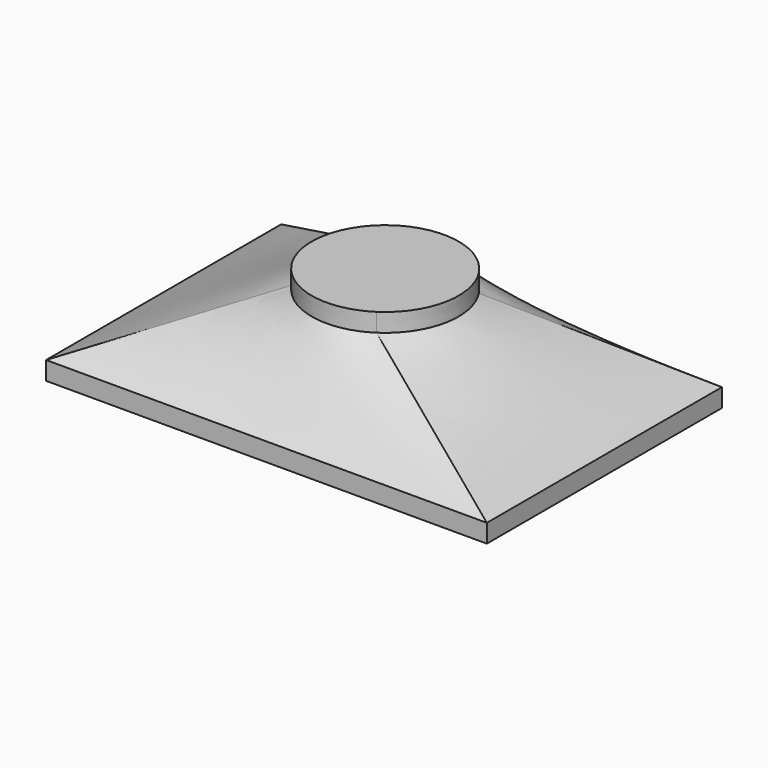
from build123d import *

# Parameters (mm, degrees)
F0_W      = 914.4
F0_H      = 609.6
F1_DEPTH  = 38.1
F1_FACE_W = 914.4
F1_FACE_H = 609.6
F5_DEPTH  = 38.1


# Not quite as in the source:
# - the arcs of a loft's sections are written as splines that run evenly, so that the points pair up as in the source's solid


with BuildPart() as f1:
    # F0 (on Top) → F1 (new body)
    with BuildSketch(Plane.XY):
        with Locations((0, -3.0270647792)):
            Rectangle(F0_W, F0_H)
    extrude(amount=F1_DEPTH)

    # F1_face (on face) → F4 section 0
    with BuildSketch(Plane(origin=(0, -3.0270647792, 38.1), x_dir=(1, 0, 0), z_dir=(0, 0, 1))):
        Rectangle(F1_FACE_W, F1_FACE_H)
    # F3 (on offset) → F4 section 1
    with BuildSketch(Plane.XY.offset(190.5)):
        with BuildLine():
            add(Edge.make_bspline(
                [(127.1917959248, 83.9524094319), (121.6971235765, 92.2770930084), (115.3826976006, 100.0604061319), (101.3563796815, 114.245945568), (93.6448345666, 120.6478211153), (77.1205669567, 131.8243905093), (68.3082530567, 136.5988079933), (49.9210540934, 144.3368980513), (40.3466236897, 147.3003792857), (20.8031031174, 151.3026195462), (10.8344962009, 152.3412796091), (-9.1142994449, 152.4538662235), (-19.0939949009, 151.5277899911), (-38.6814445909, 147.7463963189), (-48.2887144867, 144.8911723815), (-66.7620835141, 137.3611152609), (-75.6277258553, 132.6864682732), (-83.9524094319, 127.1917959248)],
                knots=[0, 0, 0, 0, 0.125, 0.125, 0.25, 0.25, 0.375, 0.375, 0.5, 0.5, 0.625, 0.625, 0.75, 0.75, 0.875, 0.875, 1, 1, 1, 1], degree=3))
            add(Edge.make_bspline(
                [(-83.9524094319, 127.1917959248), (-92.2770930084, 121.6971235765), (-100.0604061319, 115.3826976006), (-114.245945568, 101.3563796815), (-120.6478211153, 93.6448345666), (-131.8243905093, 77.1205669567), (-136.5988079933, 68.3082530567), (-144.3368980513, 49.9210540934), (-147.3003792857, 40.3466236897), (-151.3026195462, 20.8031031174), (-152.3412796091, 10.8344962009), (-152.4538662235, -9.1142994449), (-151.5277899911, -19.0939949009), (-147.7463963189, -38.6814445909), (-144.8911723815, -48.2887144867), (-137.3611152609, -66.7620835141), (-132.6864682732, -75.6277258553), (-127.1917959248, -83.9524094319)],
                knots=[0, 0, 0, 0, 0.125, 0.125, 0.25, 0.25, 0.375, 0.375, 0.5, 0.5, 0.625, 0.625, 0.75, 0.75, 0.875, 0.875, 1, 1, 1, 1], degree=3))
            add(Edge.make_bspline(
                [(-127.1917959248, -83.9524094319), (-121.6971235765, -92.2770930084), (-115.3826976006, -100.0604061319), (-101.3563796815, -114.245945568), (-93.6448345666, -120.6478211153), (-77.1205669567, -131.8243905093), (-68.3082530567, -136.5988079933), (-49.9210540934, -144.3368980513), (-40.3466236897, -147.3003792857), (-20.8031031174, -151.3026195462), (-10.8344962009, -152.3412796091), (9.1142994449, -152.4538662235), (19.0939949009, -151.5277899911), (38.6814445909, -147.7463963189), (48.2887144867, -144.8911723815), (66.7620835141, -137.3611152609), (75.6277258553, -132.6864682732), (83.9524094319, -127.1917959248)],
                knots=[0, 0, 0, 0, 0.125, 0.125, 0.25, 0.25, 0.375, 0.375, 0.5, 0.5, 0.625, 0.625, 0.75, 0.75, 0.875, 0.875, 1, 1, 1, 1], degree=3))
            add(Edge.make_bspline(
                [(83.9524094319, -127.1917959248), (92.2770930084, -121.6971235765), (100.0604061319, -115.3826976006), (114.245945568, -101.3563796815), (120.6478211153, -93.6448345666), (131.8243905093, -77.1205669567), (136.5988079933, -68.3082530567), (144.3368980513, -49.9210540934), (147.3003792857, -40.3466236897), (151.3026195462, -20.8031031174), (152.3412796091, -10.8344962009), (152.4538662235, 9.1142994449), (151.5277899911, 19.0939949009), (147.7463963189, 38.6814445909), (144.8911723815, 48.2887144867), (137.3611152609, 66.7620835141), (132.6864682732, 75.6277258553), (127.1917959248, 83.9524094319)],
                knots=[0, 0, 0, 0, 0.125, 0.125, 0.25, 0.25, 0.375, 0.375, 0.5, 0.5, 0.625, 0.625, 0.75, 0.75, 0.875, 0.875, 1, 1, 1, 1], degree=3))
        make_face()
    loft(ruled=True)

    # F5 (add): a face of the model
    f5_faces = [f1.faces().sort_by_distance(p)[0] for p in [
        (0, 0, 190.5),
    ]]
    extrude(f5_faces, amount=F5_DEPTH)


solid = f1.part
